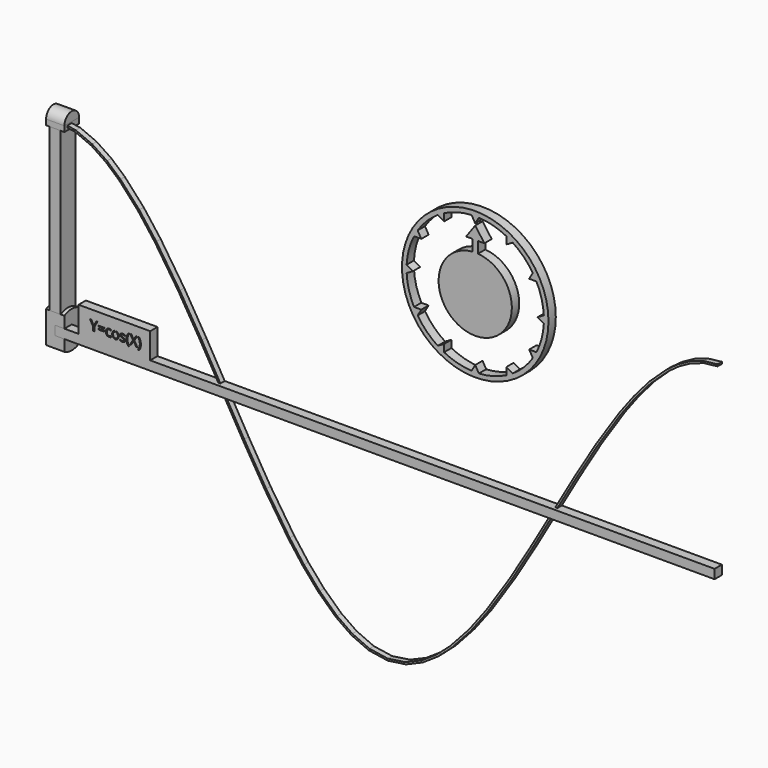
from build123d import *

# Parameters (mm, degrees)
F1_DEPTH  = 3
F3_DEPTH  = 5
F4_W      = 10
F4_H      = 3
F5_DEPTH  = 5
F7_DEPTH  = 5
F8_W      = 3.3051347101
F8_H      = 0.4867851534
F9_DEPTH  = 5
F10_R     = 40
F11_DEPTH = 5
F13_DEPTH = 3
F15_T     = -1
F17_DEPTH = 5


with BuildPart() as f1:
    # F0 (on Right) → F1 (new body, symmetric)
    with BuildSketch(Plane.YZ):
        with BuildLine():
            Line((-5, 100), (-5, 0))
            ThreePointArc((-5, 0), (0, -5), (5, 0))
            Line((5, 0), (5, 100))
            ThreePointArc((5, 100), (0, 105), (-5, 100))
        make_face()
    extrude(amount=F1_DEPTH, both=True)


with BuildPart() as f3:
    # F2 (on Right) → F3 (new body, symmetric)
    with BuildSketch(Plane.YZ):
        with BuildLine():
            Line((-5, 100), (5, 100))
            ThreePointArc((5, 100), (0, 105), (-5, 100))
        make_face()
    extrude(amount=F3_DEPTH, both=True)


with BuildPart() as f5:
    # F4 (on Right) → F5 (new body, symmetric)
    with BuildSketch(Plane.YZ):
        with Locations((0, 98.5)):
            Rectangle(F4_W, F4_H)
    extrude(amount=F5_DEPTH, both=True)


with BuildPart() as f7:
    # F6 (on Right) → F7 (new body, symmetric)
    with BuildSketch(Plane.YZ):
        with BuildLine():
            Line((-5, 8.6602540378), (-5, -8.6602540378))
            ThreePointArc((-5, -8.6602540378), (10, 0), (-5, 8.6602540378))
        make_face()
    extrude(amount=F7_DEPTH, both=True)


with BuildPart() as f9:
    # F8 (on Front) → F9 (new body)
    with BuildSketch(Plane.XZ):
        Polygon((12.7282338217, 2.5), (0, 2.5), (0, -2.5), (360, -2.5), (360, 2.5), (51.8362522125, 2.5), (51.8362522125, 16.5278445929), (12.7282338217, 16.5278445929), align=None)
        Polygon((19.6523424524, 11.6963307122), (21.0285341245, 9.097489414), (22.4138245846, 11.6963307122), (23.067799966, 11.6963307122), (21.3333435197, 8.5151669874), (21.3333435197, 6.4997854643), (20.7225873809, 6.4997854643), (20.7225873809, 8.4867332752), (18.9915429801, 11.6963307122), align=None, mode=Mode.SUBTRACT)
        with Locations((25.143460959, 8.3388779716)):
            Rectangle(F8_W, F8_H, mode=Mode.SUBTRACT)
        with BuildLine():
            add(Edge.make_bspline(
                [(30.3957362829, 6.631717889), (30.0056257511, 6.4281325094), (29.4119298396, 6.4281325094)],
                knots=[0, 0, 0, 1, 1, 1], degree=2))
            add(Edge.make_bspline(
                [(29.4119298396, 6.4281325094), (28.5657425635, 6.4281325094), (28.1017043799, 6.9490381176)],
                knots=[0, 0, 0, 1, 1, 1], degree=2))
            add(Edge.make_bspline(
                [(28.1017043799, 6.9490381176), (27.6376661962, 7.4699437257), (27.6376661962, 8.4230417598)],
                knots=[0, 0, 0, 1, 1, 1], degree=2))
            add(Edge.make_bspline(
                [(27.6376661962, 8.4230417598), (27.6376661962, 9.4000241121), (28.1090971451, 9.9334405536)],
                knots=[0, 0, 0, 1, 1, 1], degree=2))
            add(Edge.make_bspline(
                [(28.1090971451, 9.9334405536), (28.5805280939, 10.4668569952), (29.4505996883, 10.4668569952)],
                knots=[0, 0, 0, 1, 1, 1], degree=2))
            add(Edge.make_bspline(
                [(29.4505996883, 10.4668569952), (29.7315247651, 10.4668569952), (30.012449842, 10.406008851)],
                knots=[0, 0, 0, 1, 1, 1], degree=2))
            add(Edge.make_bspline(
                [(30.012449842, 10.406008851), (30.2933749189, 10.3451607068), (30.4526037074, 10.2632716156)],
                knots=[0, 0, 0, 1, 1, 1], degree=2))
            Line((30.4526037074, 10.2632716156), (30.2717652976, 9.7628382802))
            add(Edge.make_bspline(
                [(30.2717652976, 9.7628382802), (30.0761413574, 9.841315326), (29.8452596141, 9.892496008)],
                knots=[0, 0, 0, 1, 1, 1], degree=2))
            add(Edge.make_bspline(
                [(29.8452596141, 9.892496008), (29.6143778707, 9.9436766901), (29.4369515064, 9.9436766901)],
                knots=[0, 0, 0, 1, 1, 1], degree=2))
            add(Edge.make_bspline(
                [(29.4369515064, 9.9436766901), (28.2495596835, 9.9436766901), (28.2495596835, 8.4298658507)],
                knots=[0, 0, 0, 1, 1, 1], degree=2))
            add(Edge.make_bspline(
                [(28.2495596835, 8.4298658507), (28.2495596835, 7.7121989539), (28.539014874, 7.3283438388)],
                knots=[0, 0, 0, 1, 1, 1], degree=2))
            add(Edge.make_bspline(
                [(28.539014874, 7.3283438388), (28.8284700646, 6.9444887236), (29.3971443093, 6.9444887236)],
                knots=[0, 0, 0, 1, 1, 1], degree=2))
            add(Edge.make_bspline(
                [(29.3971443093, 6.9444887236), (29.8839294627, 6.9444887236), (30.3957362829, 7.1537608456)],
                knots=[0, 0, 0, 1, 1, 1], degree=2))
            Line((30.3957362829, 7.1537608456), (30.3957362829, 6.631717889))
        make_face(mode=Mode.SUBTRACT)
        with BuildLine():
            add(Edge.make_bspline(
                [(34.2007356541, 9.922635743), (34.6824027393, 9.3784144908), (34.6824027393, 8.451475472)],
                knots=[0, 0, 0, 1, 1, 1], degree=2))
            add(Edge.make_bspline(
                [(34.6824027393, 8.451475472), (34.6824027393, 7.4983774379), (34.2030103511, 6.9632549737)],
                knots=[0, 0, 0, 1, 1, 1], degree=2))
            add(Edge.make_bspline(
                [(34.2030103511, 6.9632549737), (33.7236179628, 6.4281325094), (32.8774306867, 6.4281325094)],
                knots=[0, 0, 0, 1, 1, 1], degree=2))
            add(Edge.make_bspline(
                [(32.8774306867, 6.4281325094), (32.3542503816, 6.4281325094), (31.9493543194, 6.6737997831)],
                knots=[0, 0, 0, 1, 1, 1], degree=2))
            add(Edge.make_bspline(
                [(31.9493543194, 6.6737997831), (31.5444582572, 6.9194670568), (31.3238126502, 7.377818498)],
                knots=[0, 0, 0, 1, 1, 1], degree=2))
            add(Edge.make_bspline(
                [(31.3238126502, 7.377818498), (31.1031670433, 7.8361699393), (31.1031670433, 8.451475472)],
                knots=[0, 0, 0, 1, 1, 1], degree=2))
            add(Edge.make_bspline(
                [(31.1031670433, 8.451475472), (31.1031670433, 9.4034361576), (31.5797160604, 9.9351465764)],
                knots=[0, 0, 0, 1, 1, 1], degree=2))
            add(Edge.make_bspline(
                [(31.5797160604, 9.9351465764), (32.0562650774, 10.4668569952), (32.9024523535, 10.4668569952)],
                knots=[0, 0, 0, 1, 1, 1], degree=2))
            add(Edge.make_bspline(
                [(32.9024523535, 10.4668569952), (33.7190685688, 10.4668569952), (34.2007356541, 9.922635743)],
                knots=[0, 0, 0, 1, 1, 1], degree=2))
        make_face(mode=Mode.SUBTRACT)
        with BuildLine():
            add(Edge.make_bspline(
                [(37.9864001009, 8.2058081983), (38.2297926777, 7.9499047882), (38.2297926777, 7.5620689533)],
                knots=[0, 0, 0, 1, 1, 1], degree=2))
            add(Edge.make_bspline(
                [(38.2297926777, 7.5620689533), (38.2297926777, 7.0184163754), (37.8248966154, 6.7232744424)],
                knots=[0, 0, 0, 1, 1, 1], degree=2))
            add(Edge.make_bspline(
                [(37.8248966154, 6.7232744424), (37.4200005532, 6.4281325094), (36.6875481261, 6.4281325094)],
                knots=[0, 0, 0, 1, 1, 1], degree=2))
            add(Edge.make_bspline(
                [(36.6875481261, 6.4281325094), (35.9130138048, 6.4281325094), (35.4796840304, 6.6737997831)],
                knots=[0, 0, 0, 1, 1, 1], degree=2))
            Line((35.4796840304, 6.6737997831), (35.4796840304, 7.2208644065))
            add(Edge.make_bspline(
                [(35.4796840304, 7.2208644065), (35.7606091073, 7.0786958453), (36.0819100555, 6.9973754284)],
                knots=[0, 0, 0, 1, 1, 1], degree=2))
            add(Edge.make_bspline(
                [(36.0819100555, 6.9973754284), (36.4032110037, 6.9160550114), (36.7023336564, 6.9160550114)],
                knots=[0, 0, 0, 1, 1, 1], degree=2))
            add(Edge.make_bspline(
                [(36.7023336564, 6.9160550114), (37.1640971431, 6.9160550114), (37.4126077881, 7.0633416407)],
                knots=[0, 0, 0, 1, 1, 1], degree=2))
            add(Edge.make_bspline(
                [(37.4126077881, 7.0633416407), (37.661118433, 7.2106282701), (37.661118433, 7.5131629683)],
                knots=[0, 0, 0, 1, 1, 1], degree=2))
            add(Edge.make_bspline(
                [(37.661118433, 7.5131629683), (37.661118433, 7.7406326662), (37.4643571443, 7.9021361516)],
                knots=[0, 0, 0, 1, 1, 1], degree=2))
            add(Edge.make_bspline(
                [(37.4643571443, 7.9021361516), (37.2675958557, 8.0636396371), (36.694372217, 8.2842852441)],
                knots=[0, 0, 0, 1, 1, 1], degree=2))
            add(Edge.make_bspline(
                [(36.694372217, 8.2842852441), (36.1507196391, 8.4867332752), (35.9215439185, 8.6380006243)],
                knots=[0, 0, 0, 1, 1, 1], degree=2))
            add(Edge.make_bspline(
                [(35.9215439185, 8.6380006243), (35.6923681979, 8.7892679733), (35.5803393717, 8.9809111938)],
                knots=[0, 0, 0, 1, 1, 1], degree=2))
            add(Edge.make_bspline(
                [(35.5803393717, 8.9809111938), (35.4683105455, 9.1725544143), (35.4683105455, 9.4386939608)],
                knots=[0, 0, 0, 1, 1, 1], degree=2))
            add(Edge.make_bspline(
                [(35.4683105455, 9.4386939608), (35.4683105455, 9.9152429778), (35.8561463804, 10.1910499865)],
                knots=[0, 0, 0, 1, 1, 1], degree=2))
            add(Edge.make_bspline(
                [(35.8561463804, 10.1910499865), (36.2439822152, 10.4668569952), (36.9184298694, 10.4668569952)],
                knots=[0, 0, 0, 1, 1, 1], degree=2))
            add(Edge.make_bspline(
                [(36.9184298694, 10.4668569952), (37.547383584, 10.4668569952), (38.1490409349, 10.2109535851)],
                knots=[0, 0, 0, 1, 1, 1], degree=2))
            Line((38.1490409349, 10.2109535851), (37.9386314644, 9.7309925225))
            add(Edge.make_bspline(
                [(37.9386314644, 9.7309925225), (37.3528969924, 9.9721104023), (36.8763479753, 9.9721104023)],
                knots=[0, 0, 0, 1, 1, 1], degree=2))
            add(Edge.make_bspline(
                [(36.8763479753, 9.9721104023), (36.4566663827, 9.9721104023), (36.243413541, 9.8407466518)],
                knots=[0, 0, 0, 1, 1, 1], degree=2))
            add(Edge.make_bspline(
                [(36.243413541, 9.8407466518), (36.0301606992, 9.7093829012), (36.0301606992, 9.4785011579)],
                knots=[0, 0, 0, 1, 1, 1], degree=2))
            add(Edge.make_bspline(
                [(36.0301606992, 9.4785011579), (36.0301606992, 9.3215470664), (36.1103437677, 9.2117929371)],
                knots=[0, 0, 0, 1, 1, 1], degree=2))
            add(Edge.make_bspline(
                [(36.1103437677, 9.2117929371), (36.1905268362, 9.1020388079), (36.3679532006, 9.0025208151)],
                knots=[0, 0, 0, 1, 1, 1], degree=2))
            add(Edge.make_bspline(
                [(36.3679532006, 9.0025208151), (36.5453795649, 8.9030028223), (37.0503622942, 8.714202973)],
                knots=[0, 0, 0, 1, 1, 1], degree=2))
            add(Edge.make_bspline(
                [(37.0503622942, 8.714202973), (37.7430075242, 8.4617116084), (37.9864001009, 8.2058081983)],
                knots=[0, 0, 0, 1, 1, 1], degree=2))
        make_face(mode=Mode.SUBTRACT)
        with BuildLine():
            add(Edge.make_bspline(
                [(39.1294353327, 6.7596695941), (38.8553343468, 7.5666183473), (38.8553343468, 8.4935573661)],
                knots=[0, 0, 0, 1, 1, 1], degree=2))
            add(Edge.make_bspline(
                [(38.8553343468, 8.4935573661), (38.8553343468, 9.4352819153), (39.1311413555, 10.2564475246)],
                knots=[0, 0, 0, 1, 1, 1], degree=2))
            add(Edge.make_bspline(
                [(39.1311413555, 10.2564475246), (39.4069483642, 11.0776131339), (39.9255792753, 11.6963307122)],
                knots=[0, 0, 0, 1, 1, 1], degree=2))
            Line((39.9255792753, 11.6963307122), (40.5010776109, 11.6963307122))
            add(Edge.make_bspline(
                [(40.5010776109, 11.6963307122), (39.9892707907, 11.0105095731), (39.7316613579, 10.1893439638)],
                knots=[0, 0, 0, 1, 1, 1], degree=2))
            add(Edge.make_bspline(
                [(39.7316613579, 10.1893439638), (39.474051925, 9.3681783544), (39.474051925, 8.500381457)],
                knots=[0, 0, 0, 1, 1, 1], degree=2))
            add(Edge.make_bspline(
                [(39.474051925, 8.500381457), (39.474051925, 7.64737009), (39.7373481003, 6.8335972459)],
                knots=[0, 0, 0, 1, 1, 1], degree=2))
            add(Edge.make_bspline(
                [(39.7373481003, 6.8335972459), (40.0006442756, 6.0198244017), (40.49425352, 5.3476514445)],
                knots=[0, 0, 0, 1, 1, 1], degree=2))
            Line((40.49425352, 5.3476514445), (39.9255792753, 5.3476514445))
            add(Edge.make_bspline(
                [(39.9255792753, 5.3476514445), (39.4035363187, 5.9527208409), (39.1294353327, 6.7596695941)],
                knots=[0, 0, 0, 1, 1, 1], degree=2))
        make_face(mode=Mode.SUBTRACT)
        Polygon((43.1567863336, 9.2362459297), (44.8912427799, 6.4997854643), (44.2054216408, 6.4997854643), (42.8087576958, 8.7847185794), (41.3870720841, 6.4997854643), (40.7467448846, 6.4997854643), (42.47437724, 9.2157736569), (40.863891779, 11.6963307122), (41.5326526908, 11.6963307122), (42.8224058777, 9.6377299464), (44.1235325495, 11.6963307122), (44.766134446, 11.6963307122), align=None, mode=Mode.SUBTRACT)
        with BuildLine():
            add(Edge.make_bspline(
                [(46.5085523317, 10.2513294564), (46.7826533177, 9.4284578244), (46.7826533177, 8.4935573661)],
                knots=[0, 0, 0, 1, 1, 1], degree=2))
            add(Edge.make_bspline(
                [(46.7826533177, 8.4935573661), (46.7826533177, 7.5586569079), (46.506846309, 6.7517081547)],
                knots=[0, 0, 0, 1, 1, 1], degree=2))
            add(Edge.make_bspline(
                [(46.506846309, 6.7517081547), (46.2310393003, 5.9447594014), (45.7124083892, 5.3476514445)],
                knots=[0, 0, 0, 1, 1, 1], degree=2))
            Line((45.7124083892, 5.3476514445), (45.1437341445, 5.3476514445))
            add(Edge.make_bspline(
                [(45.1437341445, 5.3476514445), (45.6373433889, 6.0164123563), (45.9006395642, 6.8318912232)],
                knots=[0, 0, 0, 1, 1, 1], degree=2))
            add(Edge.make_bspline(
                [(45.9006395642, 6.8318912232), (46.1639357395, 7.64737009), (46.1639357395, 8.500381457)],
                knots=[0, 0, 0, 1, 1, 1], degree=2))
            add(Edge.make_bspline(
                [(46.1639357395, 8.500381457), (46.1639357395, 9.3681783544), (45.9063263066, 10.1893439638)],
                knots=[0, 0, 0, 1, 1, 1], degree=2))
            add(Edge.make_bspline(
                [(45.9063263066, 10.1893439638), (45.6487168738, 11.0105095731), (45.1369100536, 11.6963307122)],
                knots=[0, 0, 0, 1, 1, 1], degree=2))
            Line((45.1369100536, 11.6963307122), (45.7124083892, 11.6963307122))
            add(Edge.make_bspline(
                [(45.7124083892, 11.6963307122), (46.2344513458, 11.0742010885), (46.5085523317, 10.2513294564)],
                knots=[0, 0, 0, 1, 1, 1], degree=2))
        make_face(mode=Mode.SUBTRACT)
        with Locations((25.143460959, 9.792409341)):
            Rectangle(F8_W, F8_H, mode=Mode.SUBTRACT)
    extrude(amount=F9_DEPTH)

    # F16 (on face) → F17 (join)
    with BuildSketch(Plane.XZ.offset(5)):
        with BuildLine():
            add(Edge.make_bspline(
                [(31.6010662604, 8.451475472), (31.6010662604, 8.7272545273), (31.6717056462, 9.1883019645), (31.8409252493, 9.4805889381), (31.9504909691, 9.602837086)],
                knots=[0, 0, 0, 0, 0.5, 1, 1, 1, 1], degree=3))
            add(Edge.make_bspline(
                [(31.7724367905, 7.5937814837), (31.6631081866, 7.820891934), (31.6010662604, 8.100786539), (31.6010662604, 8.451475472)],
                knots=[0, 0, 0, 0, 1, 1, 1, 1], degree=3))
            add(Edge.make_bspline(
                [(32.2076283062, 7.0994735762), (32.1142192072, 7.1561487598), (31.9544783266, 7.2891453977), (31.8277110506, 7.4789591804), (31.7724367905, 7.5937814837)],
                knots=[0, 0, 0, 0, 0.5, 1, 1, 1, 1], degree=3))
            add(Edge.make_bspline(
                [(32.8774306867, 6.9260317265), (32.7420032774, 6.9260317265), (32.5004890564, 6.9576007268), (32.3019392009, 7.0422512356), (32.2076283062, 7.0994735762)],
                knots=[0, 0, 0, 0, 0.5, 1, 1, 1, 1], degree=3))
            add(Edge.make_bspline(
                [(33.8321615011, 7.2954819455), (33.7209384928, 7.1713290976), (33.477096387, 6.9985420572), (33.1070151592, 6.9260317265), (32.8774306867, 6.9260317265)],
                knots=[0, 0, 0, 0, 0.5, 1, 1, 1, 1], degree=3))
            add(Edge.make_bspline(
                [(34.1845035223, 8.451475472), (34.1845035223, 8.175515292), (34.1135486879, 7.7137340595), (33.9429453228, 7.4191445508), (33.8321615011, 7.2954819455)],
                knots=[0, 0, 0, 0, 0.5, 1, 1, 1, 1], degree=3))
            add(Edge.make_bspline(
                [(33.8278926624, 9.5926482676), (33.9419580491, 9.4637691943), (34.1143745415, 9.1650719345), (34.1845035223, 8.7173344254), (34.1845035223, 8.451475472)],
                knots=[0, 0, 0, 0, 0.5, 1, 1, 1, 1], degree=3))
            add(Edge.make_bspline(
                [(33.2026399761, 9.9426417465), (33.2903249785, 9.9260537959), (33.5313056872, 9.8531234797), (33.713613178, 9.7217692435), (33.8278926624, 9.5926482676)],
                knots=[0.254073286, 0.254073286, 0.254073286, 0.254073286, 0.5, 1, 1, 1, 1], degree=3))
            Line((33.2026399761, 9.9426417465), (33.2026399761, 10.4469397426))
            add(Edge.make_bspline(
                [(32.9024523535, 10.4668569952), (33.0586753507, 10.4668569952), (33.2026399761, 10.4469397426)],
                knots=[0, 0, 0, 0.1913052842, 0.1913052842, 0.1913052842], degree=2))
            add(Edge.make_bspline(
                [(32.6001115862, 10.448417757), (32.744872609, 10.4668569952), (32.9024523535, 10.4668569952)],
                knots=[0.8137767502, 0.8137767502, 0.8137767502, 1, 1, 1], degree=2))
            Line((32.6001115862, 10.448417757), (32.6001115862, 9.945101816))
            add(Edge.make_bspline(
                [(31.9504909691, 9.602837086), (32.060461834, 9.7255372754), (32.2440540027, 9.855474242), (32.5017184949, 9.9284285371), (32.6001116816, 9.9451018322)],
                knots=[0, 0, 0, 0, 0.5, 0.7592891034, 0.7592891034, 0.7592891034, 0.7592891034], degree=3))
        make_face()
        with BuildLine():
            Line((32.6001115862, 10.6511381723), (32.6001115862, 10.448417757))
            add(Edge.make_bspline(
                [(32.6001115862, 10.448417757), (32.744872609, 10.4668569952), (32.9024523535, 10.4668569952)],
                knots=[0.8137767502, 0.8137767502, 0.8137767502, 1, 1, 1], degree=2))
            add(Edge.make_bspline(
                [(32.9024523535, 10.4668569952), (33.0586753507, 10.4668569952), (33.2026399761, 10.4469397426)],
                knots=[0, 0, 0, 0.1913052842, 0.1913052842, 0.1913052842], degree=2))
            Line((33.2026399761, 10.4469397426), (33.2026399761, 10.6511381723))
            Line((33.2026399761, 10.6511381723), (32.6001115862, 10.6511381723))
        make_face()
    extrude(amount=-F17_DEPTH)


with BuildPart() as f11:
    # F10 (on Front) → F11 (new body)
    with BuildSketch(Plane.XZ):
        with Locations((229.308500886, 92.0021682978)):
            Circle(F10_R)
        with BuildLine():
            ThreePointArc((212.308500886, 125.4274581245), (219.6027866946, 128.2243867836), (227.3182878369, 129.4493184166))
            Line((227.3182878369, 129.4493184166), (229.308500886, 126.0021682978))
            Line((229.308500886, 126.0021682978), (231.298713935, 129.4493184166))
            ThreePointArc((231.298713935, 129.4493184166), (239.0142150773, 128.2243867836), (246.308500886, 125.4274581245))
            Line((246.308500886, 125.4274581245), (246.308500886, 121.4470320264))
            Line((246.308500886, 121.4470320264), (249.7556510048, 123.4372450755))
            ThreePointArc((249.7556510048, 123.4372450755), (255.8250051805, 118.5186725923), (260.7435776637, 112.4493184166))
            Line((260.7435776637, 112.4493184166), (258.7533646146, 109.0021682978))
            Line((258.7533646146, 109.0021682978), (262.7337907127, 109.0021682978))
            ThreePointArc((262.7337907127, 109.0021682978), (265.5307193718, 101.7078824891), (266.7556510048, 93.9923813468))
            Line((266.7556510048, 93.9923813468), (263.308500886, 92.0021682978))
            Line((263.308500886, 92.0021682978), (266.7556510048, 90.0119552487))
            ThreePointArc((266.7556510048, 90.0119552487), (265.5307193718, 82.2964541064), (262.7337907127, 75.0021682978))
            Line((262.7337907127, 75.0021682978), (258.7533646146, 75.0021682978))
            Line((258.7533646146, 75.0021682978), (260.7435776637, 71.555018179))
            ThreePointArc((260.7435776637, 71.555018179), (255.8250051805, 65.4856640033), (249.7556510048, 60.5670915201))
            Line((249.7556510048, 60.5670915201), (246.308500886, 62.5573045691))
            Line((246.308500886, 62.5573045691), (246.308500886, 58.5768784711))
            ThreePointArc((246.308500886, 58.5768784711), (239.0142150773, 55.7799498119), (231.298713935, 54.555018179))
            Line((231.298713935, 54.555018179), (229.308500886, 58.0021682978))
            Line((229.308500886, 58.0021682978), (227.3182878369, 54.555018179))
            ThreePointArc((227.3182878369, 54.555018179), (219.6027866946, 55.7799498119), (212.308500886, 58.5768784711))
            Line((212.308500886, 58.5768784711), (212.308500886, 62.5573045691))
            Line((212.308500886, 62.5573045691), (208.8613507672, 60.5670915201))
            ThreePointArc((208.8613507672, 60.5670915201), (202.7919965915, 65.4856640033), (197.8734241083, 71.555018179))
            Line((197.8734241083, 71.555018179), (199.8636371573, 75.0021682978))
            Line((199.8636371573, 75.0021682978), (195.8832110592, 75.0021682978))
            ThreePointArc((195.8832110592, 75.0021682978), (193.0862824001, 82.2964541064), (191.8613507672, 90.0119552487))
            Line((191.8613507672, 90.0119552487), (195.308500886, 92.0021682978))
            Line((195.308500886, 92.0021682978), (191.8613507672, 93.9923813468))
            ThreePointArc((191.8613507672, 93.9923813468), (193.0862824001, 101.7078824891), (195.8832110592, 109.0021682978))
            Line((195.8832110592, 109.0021682978), (199.8636371573, 109.0021682978))
            Line((199.8636371573, 109.0021682978), (197.8734241083, 112.4493184166))
            ThreePointArc((197.8734241083, 112.4493184166), (202.7919965915, 118.5186725923), (208.8613507672, 123.4372450755))
            Line((208.8613507672, 123.4372450755), (212.308500886, 121.4470320264))
            Line((212.308500886, 121.4470320264), (212.308500886, 125.4274581245))
        make_face(mode=Mode.SUBTRACT)
    extrude(amount=F11_DEPTH)


with BuildPart() as f11b:
    # F10 (on Front) → F11, piece 2 (new body)
    with BuildSketch(Plane.XZ):
        with BuildLine():
            Line((227.808500886, 118.1109698415), (227.808500886, 111.9458389729))
            ThreePointArc((227.808500886, 111.9458389729), (229.308500886, 72.0021682978), (230.808500886, 111.9458389729))
            Line((230.808500886, 111.9458389729), (230.808500886, 118.1109698415))
            Line((230.808500886, 118.1109698415), (234.308500886, 118.1109698415))
            Line((234.308500886, 118.1109698415), (229.308500886, 125.0021682978))
            Line((229.308500886, 125.0021682978), (224.308500886, 118.1109698415))
            Line((224.308500886, 118.1109698415), (227.808500886, 118.1109698415))
        make_face()
    extrude(amount=F11_DEPTH)


with BuildPart() as f13:
    # F12 (on Front) → F13 (new body)
    with BuildSketch(Plane.XZ):
        Polygon((30.9103771436, 97.4506146496), (30.9103771436, -2.5493853504), (90.381167829, -2.5493853504), (90.381167829, -123.5195174813), (342.9147005081, -123.5195174813), (342.9147005081, -2.5493853504), (390.9103771436, -2.5493853504), (390.9103771436, 97.4506146496), (383.3122201436, 96.5725916496), (376.0650711436, 94.1127246496), (369.3408931436, 90.4478646496), (363.1472121436, 85.9387016496), (353.6612421436, 77.0517666496), (345.1515971436, 67.2187246496), (337.3334141436, 56.8248806496), (324.4996781436, 37.4684046496), (312.5174621436, 17.5705146496), (300.9103771436, -2.5493853504), (289.3032921436, -22.6692863504), (277.3210761436, -42.5671763504), (264.4873411436, -61.9236503504), (255.2072501436, -74.1225073504), (244.9015611436, -85.4617833504), (237.5843581436, -91.9069353504), (229.4913881436, -97.3367823504), (220.5309001436, -101.1430093504), (210.9103781436, -102.5493873504), (200.8446901436, -101.0101873504), (191.5214111436, -96.8780273504), (183.1472101436, -91.0374523504), (173.6612421436, -82.1505653504), (165.1515951436, -72.3174923504), (157.3334141436, -61.9236503504), (144.4996791436, -42.5671773504), (132.5174621436, -22.6692873504), (120.9103771436, -2.5493863504), (109.3032921436, 17.5705146496), (97.3210771436, 37.4684046496), (84.4873401436, 56.8248806496), (75.2072481436, 69.0237466496), (64.9015651436, 80.3629866496), (57.5843631436, 86.8081546496), (49.4913921436, 92.2380186496), (40.5309091436, 96.0442386496), align=None)
    extrude(amount=F13_DEPTH)


with BuildPart() as f13_1:
    # F14: moved
    add(f13.part.moved(Location((-30.9103771436, 0, 2.5493853504))))

    # F15
    f15_openings = [f13_1.faces().sort_by_distance(p)[0] for p in [
        (185.737557, -1.5, -120.970132),
        (29.735395, -1.5, 0),
        (144.605907, -3, -87.127247),
        (59.470791, -1.5, -60.485066),
        (0, -1.5, 50),
        (312.004323, -1.5, -60.485066),
        (336.002162, -1.5, 0),
        (360, -1.5, 50),
        (144.605907, 0, -87.127247),
    ]]
    offset(amount=F15_T, openings=f15_openings, kind=Kind.INTERSECTION)


solid = Compound([f1.part, f3.part, f5.part, f7.part, f9.part, f11.part, f11b.part, f13_1.part])
